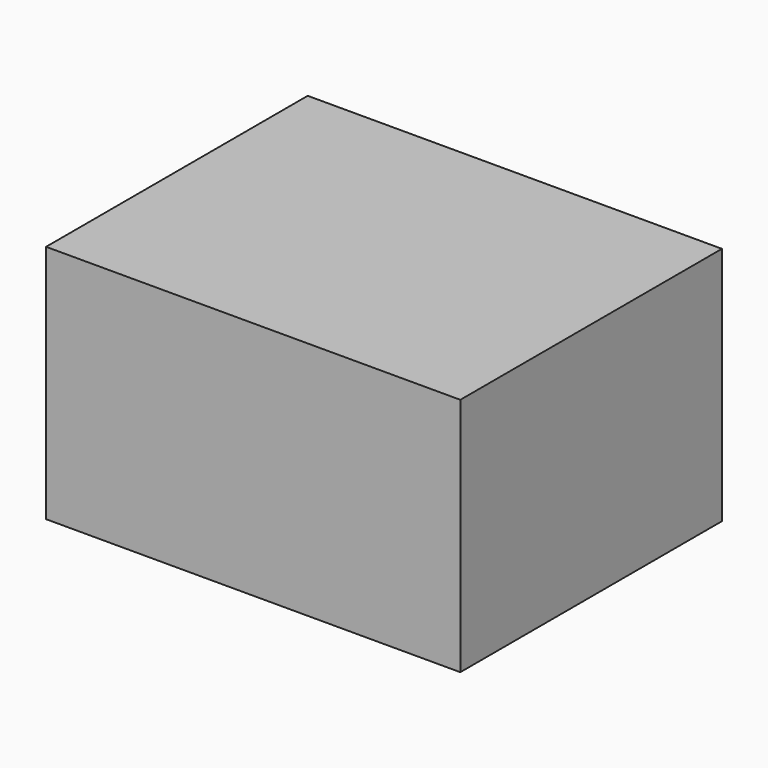
from build123d import *

# Parameters (mm, degrees)
F0_W     = 7.540625
F0_H     = 5.953125
F1_DEPTH = 4.365625


# Not quite as in the source:
# - a length typed as a fraction of an inch, garbled in the dataset ("3 / 203.2 mm" for 3/8 in), is restored


with BuildPart() as f1:
    # F0 (on Top) → F1 (new body)
    with BuildSketch(Plane.XY):
        with Locations((30.0227271199, -20.7116979659)):
            Rectangle(F0_W, F0_H)
    extrude(amount=F1_DEPTH)


solid = f1.part
